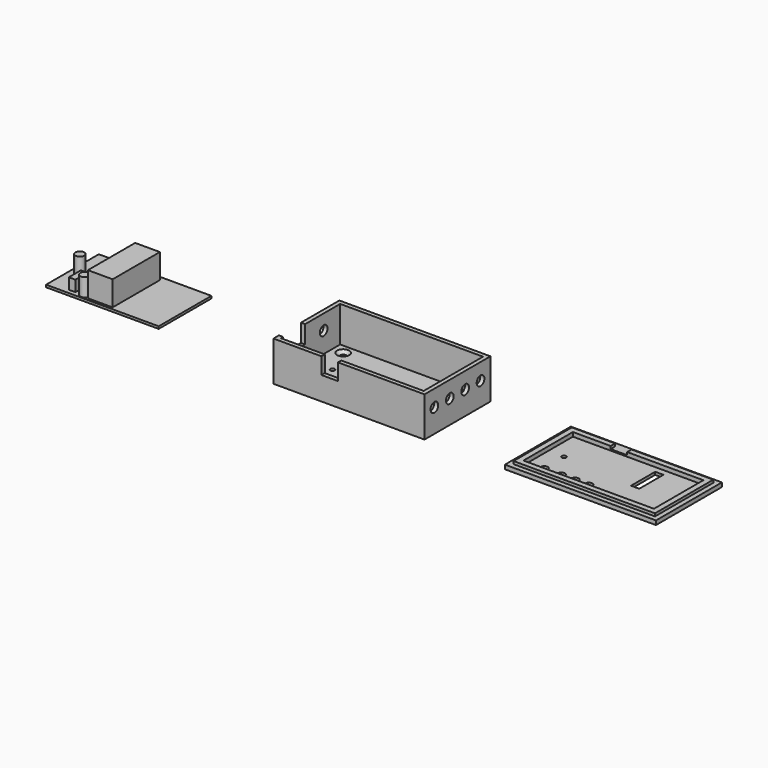
from build123d import *

# Parameters (mm, degrees)
F0_W            = 110
F0_H            = 60
F1_DEPTH        = 3
F2_W            = 110
F2_H            = 60
F2_W_2          = 104
F2_H_2          = 54
F3_DEPTH        = 24
F4_R            = 3.5
F5_DEPTH        = 25
F6_R            = 1.6
F7_DEPTH        = 25
F8_W            = 12
F8_H            = 10
F9_DEPTH        = 25
F10_R           = 3.5
F11_DEPTH       = 25
F12_DEPTH       = 2
F13_D           = 4.5
F13_CSINK_D     = 8.96
F13_CSINK_ANGLE = 90
F14_W           = 110
F14_H           = 60
F15_DEPTH       = 3
F16_R           = 1.6
F17_DEPTH       = 25
F16_W           = 103
F16_H           = 53
F18_DEPTH       = 2
F19_W           = 95
F19_H           = 45
F19_R           = 1.6
F20_DEPTH       = 3
F21_W           = 12
F21_H           = 4
F22_DEPTH       = 2
F23_R           = 2.6
F23_W           = 6
F23_H           = 22
F24_DEPTH       = 25
F25_W           = 82
F25_H           = 48
F26_DEPTH       = 1.7
F27_R           = 3.25
F28_DEPTH       = 13
F27_W           = 4.8
F27_H           = 11
F29_DEPTH       = 8
F27_W_2         = 18
F27_H_2         = 43
F30_DEPTH       = 18


# Not quite as in the source:
# - a feature names something its author has since deleted; it is built from what else it names


with BuildPart() as f1:
    # F0 (on Top) → F1 (new body)
    with BuildSketch(Plane.XY):
        with Locations((-55, -30)):
            Rectangle(F0_W, F0_H)
    extrude(amount=F1_DEPTH)

    # F2 (on face) → F3 (join)
    with BuildSketch(Plane.XY.offset(3)):
        with Locations((-55, -30)):
            Rectangle(F2_W, F2_H)
        with Locations((-55, -30)):
            Rectangle(F2_W_2, F2_H_2, mode=Mode.SUBTRACT)
    extrude(amount=F3_DEPTH)

    # F4 (on face) → F5 (cut)
    with BuildSketch(Plane(origin=(-110, 0, 0), x_dir=(0, -1, 0), z_dir=(-1, 0, 0))):
        with Locations((18, 18)):
            Circle(F4_R)
        Polygon((35, 16), (45, 16), (55, 16), (55, 27), (35, 27), align=None)
    extrude(amount=-F5_DEPTH, mode=Mode.SUBTRACT)

    # F6 (on face) → F7 (cut)
    with BuildSketch(Plane.XY.offset(3)):
        with Locations((-28, -51)):
            Circle(F6_R)
        with Locations((-28, -13)):
            Circle(F6_R)
        with Locations((-91, -30)):
            Circle(F6_R)
    extrude(amount=-F7_DEPTH, mode=Mode.SUBTRACT)

    # F8 (on face) → F9 (cut)
    with BuildSketch(Plane.XZ.offset(60)):
        with Locations((-69, 22)):
            Rectangle(F8_W, F8_H)
    extrude(amount=-F9_DEPTH, mode=Mode.SUBTRACT)

    # F10 (on face) → F11 (cut)
    with BuildSketch(Plane.YZ):
        with Locations((-51, 17)):
            Circle(F10_R)
        with Locations((-37, 17)):
            Circle(F10_R)
        with Locations((-23, 17)):
            Circle(F10_R)
        with Locations((-9, 17)):
            Circle(F10_R)
    extrude(amount=-F11_DEPTH, mode=Mode.SUBTRACT)

    # F12 (add): faces of the model
    f12_faces = [f1.faces().sort_by_distance(p)[0] for p in [
        (-61.7470035914, -58.5, 27),
        (-93.3648648649, -58.3648648649, 27),
    ]]
    extrude(f12_faces, amount=F12_DEPTH)

    # F13 (through all)
    with Locations(Plane.XY.offset(3)):
        with Locations((-99.2072820663, -10), (-99.2072820663, -50), (-14.2072820663, -50), (-14.2072820663, -10)):
            CounterSinkHole(F13_D / 2, F13_CSINK_D / 2, counter_sink_angle=F13_CSINK_ANGLE)


with BuildPart() as f15:
    # F14 (on Top) → F15 (new body)
    with BuildSketch(Plane.XY):
        with Locations((113.5470122111, -30)):
            Rectangle(F14_W, F14_H)
    extrude(amount=F15_DEPTH)

    # F16 (on face) → F17 (cut)
    with BuildSketch(Plane.XY.offset(3)):
        with Locations((77.5470122111, -30)):
            Circle(F16_R)
    extrude(amount=-F17_DEPTH, mode=Mode.SUBTRACT)

    # F16 (on face) → F18 (join)
    with BuildSketch(Plane.XY.offset(3)):
        with Locations((113.5470122111, -30)):
            Rectangle(F16_W, F16_H)
        with Locations((77.5470122111, -30)):
            Circle(F16_R, mode=Mode.SUBTRACT)
    extrude(amount=F18_DEPTH)

    # F19 (on face) → F20 (cut)
    with BuildSketch(Plane.XY.offset(5)):
        with Locations((113.5470122111, -30)):
            Rectangle(F19_W, F19_H)
        with Locations((77.5470122111, -30)):
            Circle(F19_R, mode=Mode.SUBTRACT)
    extrude(amount=-F20_DEPTH, mode=Mode.SUBTRACT)

    # F21 (on face) → F22 (cut)
    with BuildSketch(Plane.XY.offset(5)):
        with Locations((99.5470122111, -5.5)):
            Rectangle(F21_W, F21_H)
    extrude(amount=-F22_DEPTH, mode=Mode.SUBTRACT)

    # F23 (on face) → F24 (cut)
    with BuildSketch(Plane(origin=(0, 0, 0), x_dir=(1, 0, 0), z_dir=(0, 0, -1))):
        with Locations((110.0470122111, 48)):
            Circle(F23_R)
        with Locations((100.0470122111, 48)):
            Circle(F23_R)
        with Locations((90.0470122111, 48)):
            Circle(F23_R)
        with Locations((77.5470122111, 48)):
            Circle(F23_R)
        with Locations((132.5470122111, 23)):
            Rectangle(F23_W, F23_H)
    extrude(amount=-F24_DEPTH, mode=Mode.SUBTRACT)


with BuildPart() as f26:
    # F25 (on Top) → F26 (new body)
    with BuildSketch(Plane.XY):
        with Locations((-244.1147527828, -24)):
            Rectangle(F25_W, F25_H)
    extrude(amount=F26_DEPTH)

    # F27 (on face) → F28 (join)
    with BuildSketch(Plane.XY.offset(1.7)):
        with Locations((-260.112375021, -44)):
            Circle(F27_R)
        with Locations((-278.1147527828, -26)):
            Circle(F27_R)
    extrude(amount=F28_DEPTH)

    # F27 (on face) → F29 (join)
    with BuildSketch(Plane.XY.offset(1.7)):
        with Locations((-268.7147527828, -39.3)):
            Rectangle(F27_W, F27_H)
    extrude(amount=F29_DEPTH)

    # F27 (on face) → F30 (join)
    with BuildSketch(Plane.XY.offset(1.7)):
        with Locations((-247.1147527828, -24.7)):
            Rectangle(F27_W_2, F27_H_2)
    extrude(amount=F30_DEPTH)


solid = Compound([f1.part, f15.part, f26.part])
